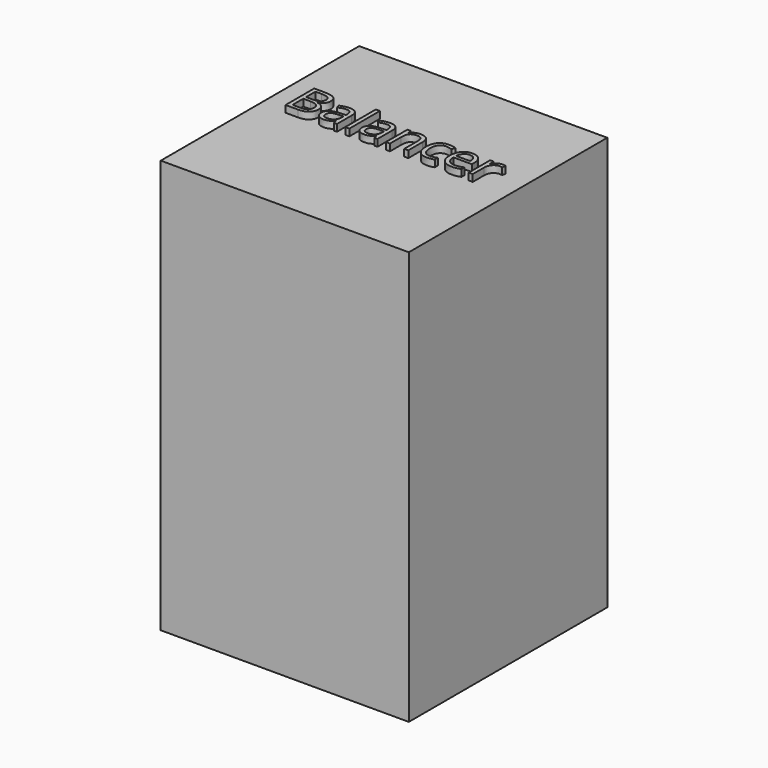
from build123d import *

# Parameters (mm, degrees)
F0_W         = 914.4
F0_H         = 914.4
F1_DEPTH     = 1524
F2_TEXT_SIZE = 184.8182817296
F3_DEPTH     = 25.4


# Not quite as in the source:
# - Text() gives the source's letters only with a copy of the font that has no kerning and outlines rounded to 1/6400 em; it was checked with that copy


with BuildPart() as f1:
    # F0 (on Top) → F1 (new body)
    with BuildSketch(Plane.XY):
        Rectangle(F0_W, F0_H)
    extrude(amount=F1_DEPTH)

    # F2 (on face) → F3 (join)
    with BuildSketch(Plane.XY.offset(1524)):
        with Locations((-381, 0)):
            Text('Balancer', F2_TEXT_SIZE, font='Open Sans', text_align=(TextAlign.LEFT, TextAlign.BOTTOM))
    extrude(amount=F3_DEPTH)


solid = f1.part
